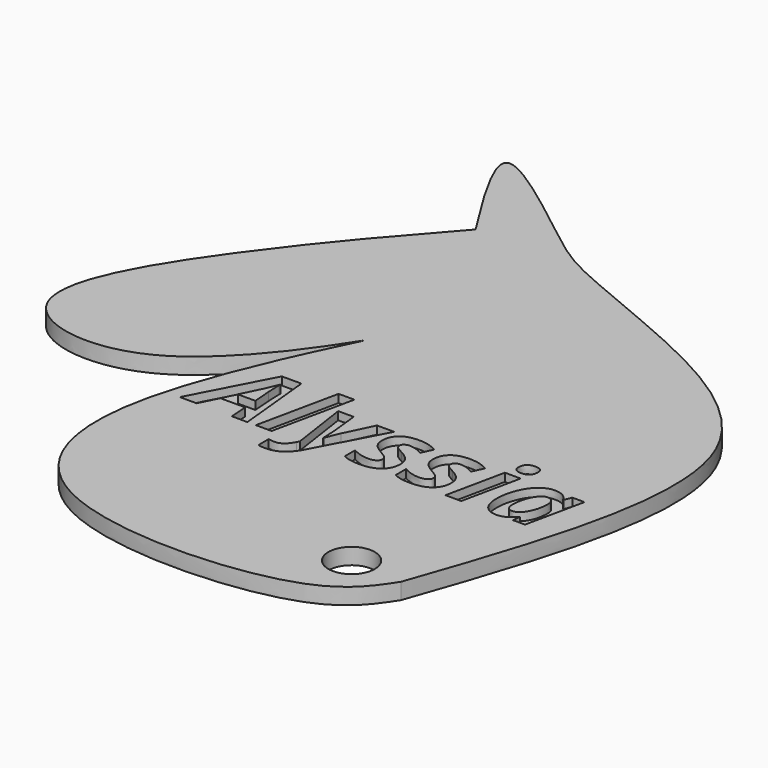
from build123d import *

# Parameters (mm, degrees)
F0_R         = 2.8558299551
F1_DEPTH     = 2
F2_TEXT_SIZE = 13.2780082988
F3_DEPTH     = 1


# Not quite as in the source:
# - Text() gives the source's letters only with a copy of the font that has no kerning and outlines rounded to 1/6400 em; it was checked with that copy


with BuildPart() as f1:
    # F0 (on Top) → F1 (new body)
    with BuildSketch(Plane.XY):
        with BuildLine():
            add(Edge.make_bspline(
                [(-26.8034636974, 47.6769581437), (-31.0622305448, 54.3256153484), (-38.1746507128, 66.2827529352), (-19.169704934, 51.055802087), (-14.1387155938, 47.4653533516), (0.5069513485, 41.8833845934), (28.2068368232, 28.3338365521), (19.0037212025, 1.4453727953), (13.5203338848, -14.2319248136)],
                knots=[0, 0, 0, 0, 0.1463319136, 0.298606348, 0.4062806405, 0.556498274, 0.7512995489, 1, 1, 1, 1], degree=3))
            add(Edge.make_bspline(
                [(-26.8034636974, 47.6769581437), (-31.7286497931, 42.1076506276), (-41.2814438672, 31.305531316), (-56.0435255491, 7.6137827464), (-32.0928276551, 3.051134261), (-14.3470042449, 34.396352715), (-33.8007517813, -1.7703824172), (-27.172899948, -24.2839051699), (7.9478512452, -22.7210015285), (12.058032038, -16.4595840744), (13.5203338848, -14.2319248136)],
                knots=[0, 0, 0, 0, 0.1359263086, 0.2636399946, 0.3742309139, 0.4981579981, 0.6364907837, 0.7636275887, 0.9159044745, 1, 1, 1, 1], degree=3))
        make_face()
        with Locations((7.0283240639, -13.738417998)):
            Circle(F0_R, mode=Mode.SUBTRACT)
    extrude(amount=F1_DEPTH)

    # F2 (on face) → F3 (cut)
    with BuildSketch(Plane.XY.offset(2)):
        with Locations((-26.3994239635, 2.5516381682)):
            Text('Alyssia', F2_TEXT_SIZE, font='Open Sans', font_style=FontStyle.BOLDITALIC, text_align=(TextAlign.LEFT, TextAlign.BOTTOM))
    extrude(amount=-F3_DEPTH, mode=Mode.SUBTRACT)


solid = f1.part
